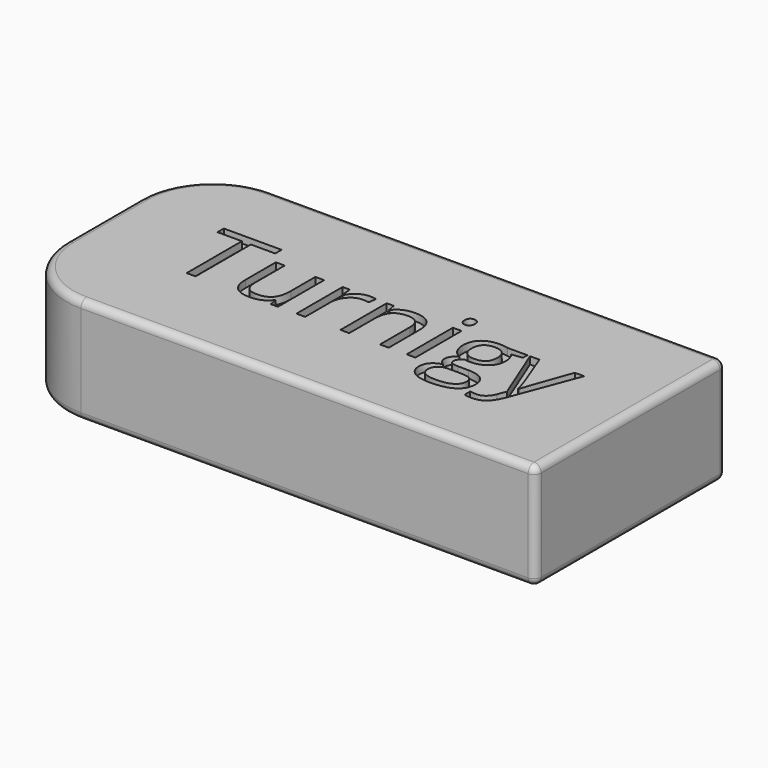
from build123d import *

# Parameters (mm, degrees)
F0_W         = 72.5
F0_H         = 32.7
F1_DEPTH     = 7.3
F2_R         = 10
F3_R         = 1
F4_TEXT_SIZE = 14.8285699731
F5_DEPTH     = 1


# Not quite as in the source:
# - Text() gives the source's letters only with a copy of the font that has no kerning and outlines rounded to 1/6400 em; it was checked with that copy


with BuildPart() as f1:
    # F0 (on Top) → F1 (new body, symmetric)
    with BuildSketch(Plane.XY):
        Rectangle(F0_W, F0_H)
    extrude(amount=F1_DEPTH, both=True)

    # F2
    f2_edges = [f1.edges().sort_by_distance(p)[0] for p in [
        (-36.25, 16.35, 0),
        (-36.25, -16.35, 0),
    ]]
    fillet(f2_edges, radius=F2_R)

    # F3
    f3_edges = [f1.edges().sort_by_distance(p)[0] for p in [
        (5, 16.35, 7.3),
        (-33.321068, 13.421068, 7.3),
        (36.25, 0, 7.3),
        (-36.25, 0, 7.3),
        (5, -16.35, 7.3),
        (-33.321068, -13.421068, 7.3),
        (5, 16.35, -7.3),
        (-33.321068, 13.421068, -7.3),
        (36.25, 0, -7.3),
        (-36.25, 0, -7.3),
        (5, -16.35, -7.3),
        (-33.321068, -13.421068, -7.3),
        (36.25, 16.35, 0),
        (36.25, -16.35, 0),
    ]]
    fillet(f3_edges, radius=F3_R)

    # F4 (on face) → F5 (cut)
    with BuildSketch(Plane.XY.offset(7.3)):
        with Locations((-24.8111995339, -4.3265703806)):
            Text('Turnigy', F4_TEXT_SIZE, font='Open Sans', text_align=(TextAlign.LEFT, TextAlign.BOTTOM))
    extrude(amount=-F5_DEPTH, mode=Mode.SUBTRACT)


solid = f1.part
